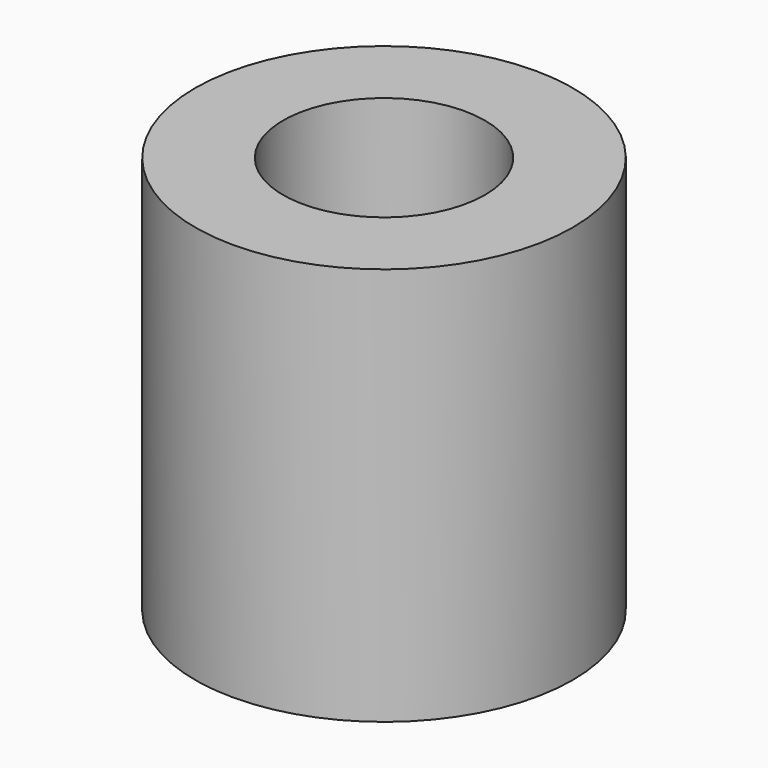
from build123d import *

# Parameters (mm, degrees)
F0_R     = 9.1481324812
F0_R_2   = 4.8908401844
F2_DEPTH = 17.78
F3_R     = 9.1481324812
F3_R_2   = 4.5098401844
F4_DEPTH = 1.524


# Not quite as in the source:
# - the program builds the solid bodies; features that only make, move or delete a surface that nothing else refers to are left out


with BuildPart() as f2:
    # F0 (on Top) → F2 (new body)
    with BuildSketch(Plane.XY):
        Circle(F0_R)
        Circle(F0_R_2, mode=Mode.SUBTRACT)
    extrude(amount=F2_DEPTH)

    # F3 (on face) → F4 (join)
    with BuildSketch(Plane(origin=(0, 0, 0), x_dir=(1, 0, 0), z_dir=(0, 0, -1))):
        Circle(F3_R)
        Circle(F3_R_2, mode=Mode.SUBTRACT)
    extrude(amount=F4_DEPTH)


solid = f2.part
